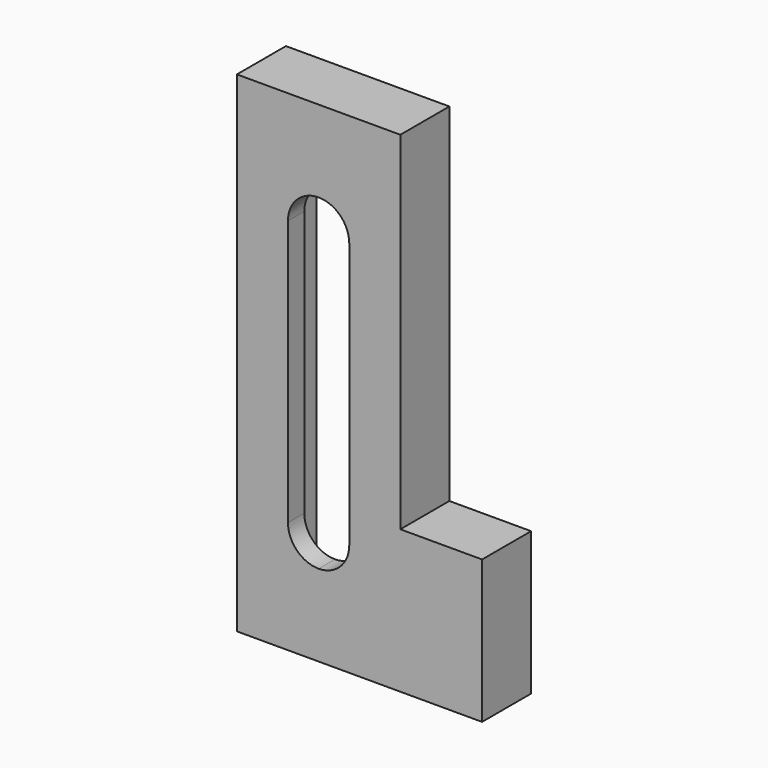
from build123d import *

# Parameters (mm, degrees)
F0_W     = 25
F0_H     = 100
F0_W_2   = 15
F0_H_2   = 80
F1_DEPTH = 15
F2_DEPTH = 10
F3_R     = 7.49999


# Not quite as in the source:
# - a fillet or chamfer is up to 0.001 mm smaller than in the source, because OpenCascade refuses the exact size


with BuildPart() as f1:
    # F0 (on Front) → F1 (new body)
    with BuildSketch(Plane.XZ):
        Polygon((20, -25), (20, 60), (-20, 60), (-20, -60), (40, -60), (40, -25), align=None)
        Rectangle(F0_W, F0_H, mode=Mode.SUBTRACT)
        Rectangle(F0_W, F0_H)
        Rectangle(F0_W_2, F0_H_2, mode=Mode.SUBTRACT)
    extrude(amount=F1_DEPTH)

    # F0 (on Front) → F2 (cut)
    with BuildSketch(Plane.XZ):
        Rectangle(F0_W, F0_H)
        Rectangle(F0_W_2, F0_H_2, mode=Mode.SUBTRACT)
    extrude(amount=F2_DEPTH, mode=Mode.SUBTRACT)

    # F3 (radius 7.5 in the source; OpenCascade refuses exactly that, so slightly less here)
    f3_edges = [f1.edges().sort_by_distance(p)[0] for p in [
        (7.5, -12.5, 40),
        (-7.5, -12.5, 40),
        (-7.5, -12.5, -40),
        (7.5, -12.5, -40),
    ]]
    fillet(f3_edges, radius=F3_R)


solid = f1.part
